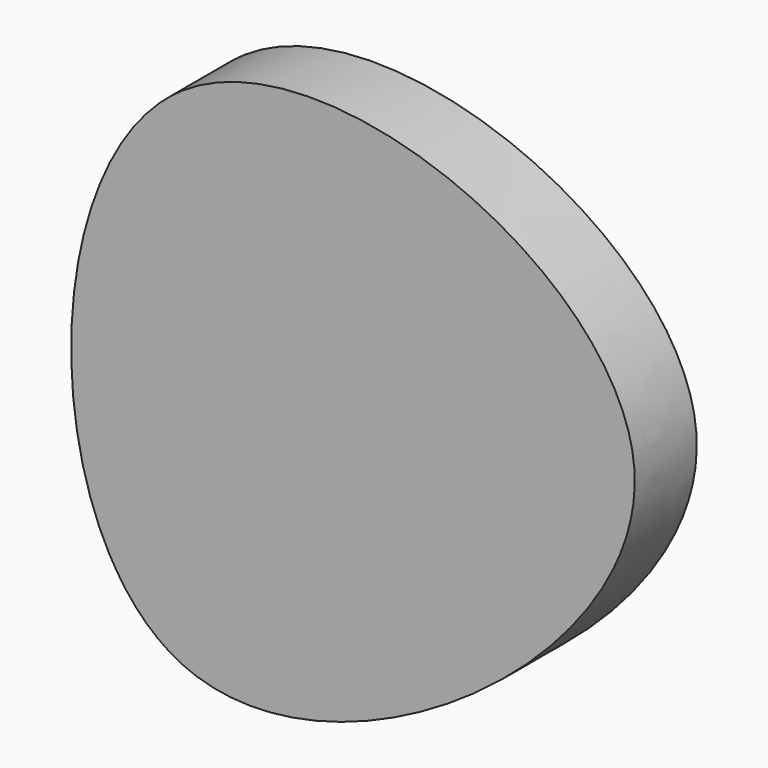
from build123d import *
from build123d import SkipClean  # not in build123d's __all__

# Parameters (mm, degrees)
F1_DEPTH = 8.89
F2_T     = -2.54
F3_R     = 3.175
F4_DEPTH = 60.452
F5_R     = 3.175
F6_DEPTH = 25.4
F7_DEPTH = 25.4


with BuildPart() as f1:
    # F0 (on Front) → F1 (new body)
    with BuildSketch(Plane.XZ):
        with BuildLine():
            add(Edge.make_bspline(
                [(0, 57.8966848552), (16.8692985273, 69.3906885455), (86.5998771546, 39.9030745477), (-16.4315827867, -32.0723852166), (-17.1297697278, 46.2252074582), (0, 57.8966848552)],
                knots=[0, 0, 0, 0, 0.3249199494, 0.6700631088, 1, 1, 1, 1], degree=3))
        make_face()
    extrude(amount=F1_DEPTH)

    # F2
    f2_openings = [f1.faces().sort_by_distance(p)[0] for p in [
        (17.417894, 0, 31.001503),
    ]]
    offset(amount=F2_T, openings=f2_openings, kind=Kind.INTERSECTION)

    # F3 (on Top) → F4 (join)
    with BuildSketch(Plane.XY):
        Polygon((8.5129914572, 0), (8.5129914572, -7.9817892178), (16.2699775716, -7.9828979896), (16.2699775716, 0), align=None)
        with Locations((12.3914845144, -3.97121749)):
            Circle(F3_R, mode=Mode.SUBTRACT)
    with SkipClean():  # cleaning this boolean's faces spoils the solid; the shape is the same uncleaned
        extrude(amount=F4_DEPTH)

    # F5 (on Top) → F6 (cut)
    with BuildSketch(Plane.XY):
        with Locations((12.3739881644, -3.4136278776)):
            Circle(F5_R)
    extrude(amount=F6_DEPTH, mode=Mode.SUBTRACT)

    # F5 (on Top) → F7 (cut)
    with BuildSketch(Plane.XY):
        with Locations((12.3739881644, -3.4136278776)):
            Circle(F5_R)
    extrude(amount=-F7_DEPTH, mode=Mode.SUBTRACT)


solid = f1.part
